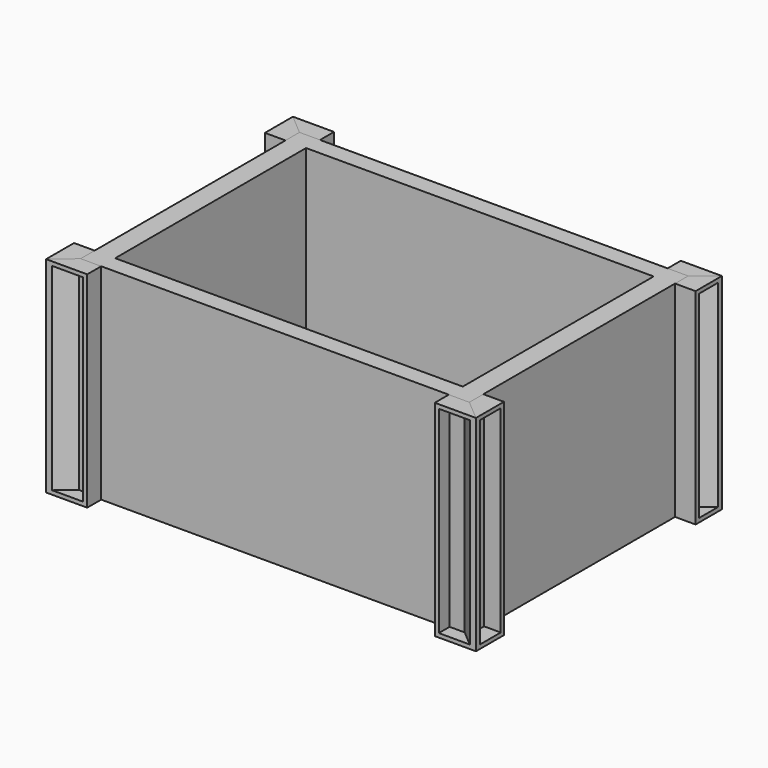
from build123d import *

# Parameters (mm, degrees)
F0_W     = 66.6093081236
F0_H     = 45.7200035453
F1_DEPTH = 1.524
F0_W_2   = 3.9413794875
F0_H_2   = 45.71999982
F0_H_3   = 3.1531043351
F0_H_4   = 3.3501740545
F0_H_5   = 3.3501703292
F2_DEPTH = 39.37
F3_DEPTH = 39.37
F4_DEPTH = 39.37
F5_T     = -0.762
F5_2_T   = -0.762
F5_3_T   = -0.762
F5_4_T   = -0.762
F5_5_T   = -0.762
F5_6_T   = -0.762
F5_7_T   = -0.762
F5_8_T   = -0.762


# Not quite as in the source:
# - ends of sketch curves that miss each other by under 0.0002 mm in the source are joined


with BuildPart() as f1:
    # F0 (on Top) → F1 (new body)
    with BuildSketch(Plane.XY):
        Rectangle(F0_W, F0_H)
    extrude(amount=F1_DEPTH)

    # F0 (on Top) → F2 (join)
    with BuildSketch(Plane.XY):
        Polygon((33.3046540618, -26.2101721019), (33.3046540618, -22.8599980474), (-33.3046540618, -22.8600017726), (-33.3046540618, -26.2101721019), align=None)
        with Locations((-35.2753438056, 1.8626e-06)):
            Rectangle(F0_W_2, F0_H_2)
        with Locations((35.2753438056, 24.6336199343)):
            Rectangle(F0_W_2, F0_H_3)
        Polygon((33.3046540618, 22.8600017726), (33.3046540618, -22.8600017726), (37.2460335493, -22.8599980474), (37.2460335493, 23.0570677668), (33.3046540618, 23.0570677668), (33.3046540618, 26.2101721019), (-33.3046540618, 26.2101721019), (-33.3046540618, 22.8600017726), align=None)
        with Locations((35.2753438056, -24.5350850746)):
            Rectangle(F0_W_2, F0_H_4)
        with Locations((-35.2753438056, -24.5350850746)):
            Rectangle(F0_W_2, F0_H_4)
        with Locations((-35.2753438056, 24.5350869372)):
            Rectangle(F0_W_2, F0_H_5)
    extrude(amount=F2_DEPTH)


with BuildPart() as f3:
    # F0 (on Top) → F3 (new body)
    with BuildSketch(Plane.XY):
        Polygon((-41.1874130368, 22.8600017726), (-37.2460335493, 22.8600017726), (-37.2460335493, 26.2101721019), (-41.1874130368, 29.5603424311), align=None)
    extrude(amount=F3_DEPTH)

    # F5#8
    f5_8_openings = [f3.faces().sort_by_distance(p)[0] for p in [
        (-41.187413, 26.210172, 19.685),
    ]]
    offset(amount=F5_8_T, openings=f5_8_openings)


with BuildPart() as f3b:
    # F0 (on Top) → F3, piece 2 (new body)
    with BuildSketch(Plane.XY):
        Polygon((-33.3046540618, -29.5603461564), (-33.3046540618, -26.2101721019), (-37.2460335493, -26.2101721019), (-41.1874130368, -29.5603461564), align=None)
    extrude(amount=F3_DEPTH)

    # F5
    f5_openings = [f3b.faces().sort_by_distance(p)[0] for p in [
        (-37.246034, -29.560346, 19.685),
    ]]
    offset(amount=F5_T, openings=f5_openings)


with BuildPart() as f3c:
    # F0 (on Top) → F3, piece 3 (new body)
    with BuildSketch(Plane.XY):
        Polygon((41.1874130368, -22.8599980474), (37.2460335493, -22.8599980474), (37.2460335493, -26.2101721019), (41.1874130368, -29.5603461564), align=None)
    extrude(amount=F3_DEPTH)

    # F5#3
    f5_3_openings = [f3c.faces().sort_by_distance(p)[0] for p in [
        (41.187413, -26.210172, 19.685),
    ]]
    offset(amount=F5_3_T, openings=f5_3_openings)


with BuildPart() as f3d:
    # F0 (on Top) → F3, piece 4 (new body)
    with BuildSketch(Plane.XY):
        Polygon((37.2460335493, 26.2101721019), (37.2460335493, 23.0570677668), (41.1874130368, 23.0570677668), (41.1874130368, 29.3632764369), align=None)
    extrude(amount=F3_DEPTH)

    # F5#4
    f5_4_openings = [f3d.faces().sort_by_distance(p)[0] for p in [
        (41.187413, 26.210172, 19.685),
    ]]
    offset(amount=F5_4_T, openings=f5_4_openings)


with BuildPart() as f4:
    # F0 (on Top) → F4 (new body)
    with BuildSketch(Plane.XY):
        Polygon((-37.2460335493, 26.2101721019), (-33.3046540618, 26.2101721019), (-33.3046540618, 29.5603424311), (-41.1874130368, 29.5603424311), align=None)
    extrude(amount=F4_DEPTH)

    # F5#6
    f5_6_openings = [f4.faces().sort_by_distance(p)[0] for p in [
        (-37.246034, 29.560342, 19.685),
    ]]
    offset(amount=F5_6_T, openings=f5_6_openings)


with BuildPart() as f4b:
    # F0 (on Top) → F4, piece 2 (new body)
    with BuildSketch(Plane.XY):
        Polygon((-37.2460335493, -26.2101721019), (-37.2460335493, -22.8599980474), (-41.1874130368, -22.8599980474), (-41.1874130368, -29.5603461564), align=None)
    extrude(amount=F4_DEPTH)

    # F5#7
    f5_7_openings = [f4b.faces().sort_by_distance(p)[0] for p in [
        (-41.187413, -26.210172, 19.685),
    ]]
    offset(amount=F5_7_T, openings=f5_7_openings)


with BuildPart() as f4c:
    # F0 (on Top) → F4, piece 3 (new body)
    with BuildSketch(Plane.XY):
        Polygon((37.2460335493, -26.2101721019), (33.3046540618, -26.2101721019), (33.3046540618, -29.5603461564), (41.1874130368, -29.5603461564), align=None)
    extrude(amount=F4_DEPTH)

    # F5#2
    f5_2_openings = [f4c.faces().sort_by_distance(p)[0] for p in [
        (37.246034, -29.560346, 19.685),
    ]]
    offset(amount=F5_2_T, openings=f5_2_openings, kind=Kind.INTERSECTION)


with BuildPart() as f4d:
    # F0 (on Top) → F4, piece 4 (new body)
    with BuildSketch(Plane.XY):
        Polygon((33.3046540618, 26.2101721019), (37.2460335493, 26.2101721019), (41.1874130368, 29.3632764369), (33.3046540618, 29.3632764369), align=None)
    extrude(amount=F4_DEPTH)

    # F5#5
    f5_5_openings = [f4d.faces().sort_by_distance(p)[0] for p in [
        (37.246034, 29.363276, 19.685),
    ]]
    offset(amount=F5_5_T, openings=f5_5_openings)


solid = Compound([f1.part, f3.part, f3b.part, f3c.part, f3d.part, f4.part, f4b.part, f4c.part, f4d.part])
